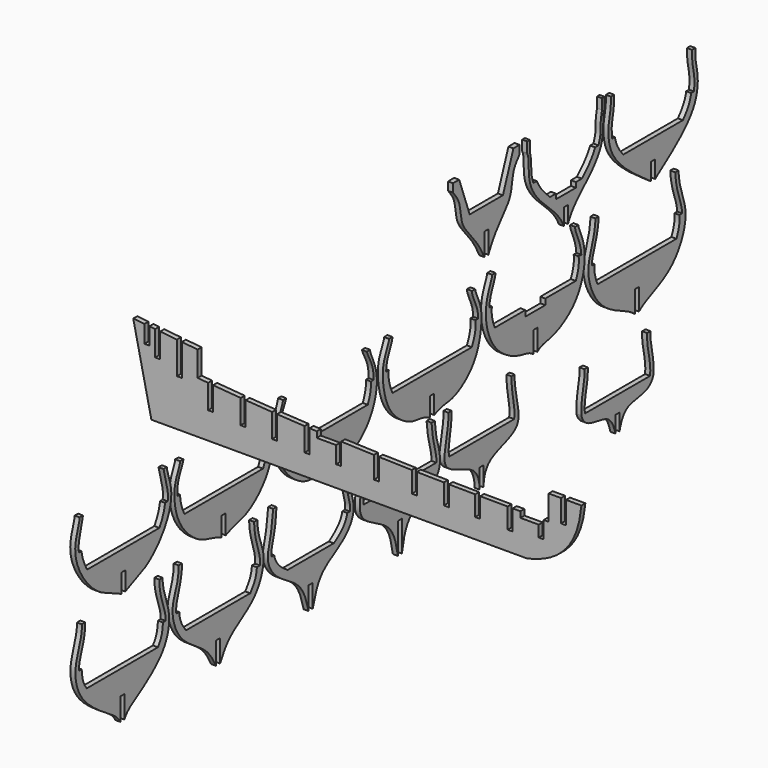
from build123d import *

# Parameters (mm, degrees)
F2_DEPTH = 6
F3_DEPTH = 6
F4_DEPTH = 6


# Not quite as in the source:
# - the dataset's text gives a spline's control points without its knots; the knots are read off the source's solid


with BuildPart() as f2:
    # F1 (on Front) → F2 (new body)
    with BuildSketch(Plane.XZ):
        with BuildLine():
            Line((-52.7647346169, 6.4092771036), (-52.7647346169, 27.4262808222))
            Line((-52.7647346169, 27.4262808222), (-66.1979233911, 28.7622259646))
            Line((-66.1979233911, 28.7622259646), (-44.4009490311, -71.2377740354))
            Line((-44.4009490311, -71.2377740354), (406.4361155033, -71.2503492832))
            add(Edge.make_bspline(
                [(472.4627340883, 6.0305400733), (469.2855259031, -29.0932188761), (455.8456540108, -61.0640123487), (406.4361155033, -71.2503492832)],
                knots=[0, 0, 0, 0, 101.6457093118, 101.6457093118, 101.6457093118, 101.6457093118], degree=3))
            Line((472.4627340883, 6.0305400733), (453.9572103575, 6.0305400733))
            Line((453.9572103575, 6.0305400733), (453.9572103575, -20.8669396024))
            Line((453.9572103575, -20.8669396024), (447.9572103575, -20.8669396024))
            Line((447.9572103575, -20.8669396024), (447.9572103575, 6.0305400733))
            Line((447.9572103575, 6.0305400733), (433.1729027743, 6.0305400733))
            Line((433.1729027743, 6.0305400733), (433.1729027743, -23.9694599267))
            Line((433.1729027743, -23.9694599267), (427.1729027743, -23.9694599267))
            Line((427.1729027743, -23.9694599267), (427.1729027743, -44.4963090949))
            Line((427.1729027743, -44.4963090949), (421.1729027743, -44.4963090949))
            Line((421.1729027743, -44.4963090949), (421.1729027743, -30.8844919416))
            Line((421.1729027743, -30.8844919416), (399.1729027743, -30.8844919416))
            Line((399.1729027743, -30.8844919416), (399.1729027743, -23.8844919416))
            add(Edge.make_bspline(
                [(389.837728412, -23.8556215321), (392.9609048209, -23.8660342773), (396.0726119054, -23.8755794708), (399.1729027743, -23.8844919416)],
                knots=[372.875417635, 372.875417635, 372.875417635, 372.875417635, 383.3713742335, 383.3713742335, 383.3713742335, 383.3713742335], degree=3))
            Line((389.837728412, -23.8556215321), (389.837728412, -48.3556215321))
            Line((389.837728412, -48.3556215321), (383.837728412, -48.3556215321))
            Line((383.837728412, -48.3556215321), (383.837728412, -23.8345407252))
            add(Edge.make_bspline(
                [(350.769388437, -23.667134025), (361.9320358553, -23.7417108378), (372.9540771428, -23.7942467699), (383.837728412, -23.8345407252)],
                knots=[329.7645780584, 329.7645780584, 329.7645780584, 329.7645780584, 366.1698310192, 366.1698310192, 366.1698310192, 366.1698310192], degree=3))
            Line((350.769388437, -23.667134025), (350.769388437, -47.6760274548))
            Line((350.769388437, -47.6760274548), (344.769388437, -47.6760274548))
            Line((344.769388437, -47.6760274548), (344.769388437, -23.6249695371))
            add(Edge.make_bspline(
                [(313.1183860302, -23.3244343777), (323.79185462, -23.4504439584), (334.3415946227, -23.5479952891), (344.769388437, -23.6249695371)],
                knots=[289.4005992863, 289.4005992863, 289.4005992863, 289.4005992863, 323.2565547842, 323.2565547842, 323.2565547842, 323.2565547842], degree=3))
            Line((313.1183860302, -23.3244343777), (313.1183860302, -47.6760274548))
            Line((313.1183860302, -47.6760274548), (307.1183860302, -47.6760274548))
            Line((307.1183860302, -47.6760274548), (307.1183860302, -23.2507163116))
            add(Edge.make_bspline(
                [(274.6596933386, -22.7436511652), (285.6039372317, -22.9476874536), (296.4229113646, -23.114099956), (307.1183860302, -23.2507163116)],
                knots=[249.2912534765, 249.2912534765, 249.2912534765, 249.2912534765, 283.0703857381, 283.0703857381, 283.0703857381, 283.0703857381], degree=3))
            Line((274.6596933386, -22.7436511652), (274.6596933386, -47.7436511652))
            Line((274.6596933386, -47.7436511652), (268.6600744313, -47.6760274548))
            Line((268.6600744313, -47.6760274548), (268.6600744313, -22.6282312507))
            add(Edge.make_bspline(
                [(229.0721806654, -21.6760274548), (242.4463483489, -22.0569030554), (255.6413320048, -22.3699669668), (268.6600744313, -22.6282312507)],
                knots=[203.116799722, 203.116799722, 203.116799722, 203.116799722, 243.1315638336, 243.1315638336, 243.1315638336, 243.1315638336], degree=3))
            Line((229.0721806654, -21.6760274548), (229.0721806654, -47.6760274548))
            Line((229.0721806654, -47.6760274548), (223.0721806654, -47.6760274548))
            Line((223.0721806654, -47.6760274548), (223.0721806654, -21.5009235146))
            add(Edge.make_bspline(
                [(183.718174545, -20.1332325707), (197.0050074387, -20.6617902502), (210.122129551, -21.1137964867), (223.0721806654, -21.5009235146)],
                knots=[158.5535490267, 158.5535490267, 158.5535490267, 158.5535490267, 197.1448620341, 197.1448620341, 197.1448620341, 197.1448620341], degree=3))
            Line((183.718174545, -20.1332325707), (183.718174545, -46.1332325707))
            Line((183.718174545, -46.1332325707), (177.718174545, -46.1332325707))
            Line((177.718174545, -46.1332325707), (177.718174545, -25.8504879718))
            Line((177.718174545, -25.8504879718), (154.3836850367, -25.8504879718))
            Line((154.3836850367, -25.8504879718), (154.3836850367, -18.8504879718))
            add(Edge.make_bspline(
                [(145.7038573316, -18.4253957008), (148.6049499698, -18.5710339991), (151.4982173473, -18.7126937317), (154.3836850367, -18.8504879718)],
                knots=[122.1894396031, 122.1894396031, 122.1894396031, 122.1894396031, 130.4161202076, 130.4161202076, 130.4161202076, 130.4161202076], degree=3))
            Line((145.7038573316, -18.4253957008), (145.7038573316, -46.1190585614))
            Line((145.7038573316, -46.1190585614), (139.7038573316, -46.1190585614))
            Line((139.7038573316, -46.1190585614), (139.7038573316, -18.1190585614))
            add(Edge.make_bspline(
                [(106.7340095181, -16.2487908881), (117.8343414661, -16.9327762992), (128.8238460829, -17.5542327451), (139.7038573316, -18.1190585614)],
                knots=[85.7901099469, 85.7901099469, 85.7901099469, 85.7901099469, 116.5285186795, 116.5285186795, 116.5285186795, 116.5285186795], degree=3))
            Line((106.7340095181, -16.2487908881), (106.7340095181, -44.4963090949))
            Line((106.7340095181, -44.4963090949), (100.7340095181, -44.4963090949))
            Line((100.7340095181, -44.4963090949), (100.7340095181, -15.8736411522))
            add(Edge.make_bspline(
                [(68.9865160879, -13.7047010206), (79.668117991, -14.4872744185), (90.2502452137, -15.2086158496), (100.7340095181, -15.8736411522)],
                knots=[51.3347121322, 51.3347121322, 51.3347121322, 51.3347121322, 80.2617577764, 80.2617577764, 80.2617577764, 80.2617577764], degree=3))
            Line((68.9865160879, -13.7047010206), (68.9865160879, -42.2594336062))
            Line((68.9865160879, -42.2594336062), (62.9865160879, -42.2594336062))
            Line((62.9865160879, -42.2594336062), (62.9865160879, -13.2594336062))
            add(Edge.make_bspline(
                [(29.770050062, -10.5860133059), (40.9473587591, -11.5457307631), (52.0191171292, -12.4351155869), (62.9865160879, -13.2594336062)],
                knots=[16.3300220537, 16.3300220537, 16.3300220537, 16.3300220537, 45.9278927601, 45.9278927601, 45.9278927601, 45.9278927601], degree=3))
            Line((29.770050062, -10.5860133059), (29.770050062, -39.0649404954))
            Line((29.770050062, -39.0649404954), (23.770050062, -39.0649404954))
            Line((23.770050062, -39.0649404954), (23.770050062, -10.0649404954))
            add(Edge.make_bspline(
                [(11.1729027743, -8.9323863213), (15.3867154839, -9.3200080517), (19.5857439628, -9.6974349483), (23.770050062, -10.0649404954)],
                knots=[0, 0, 0, 0, 11.0428828538, 11.0428828538, 11.0428828538, 11.0428828538], degree=3))
            Line((11.1729027743, -8.9323863213), (11.1729027743, 21.0676136787))
            Line((11.1729027743, 21.0676136787), (-7.7765522316, 22.95215746))
            Line((-7.7765522316, 22.95215746), (-7.7765522316, -15.2084504512))
            Line((-7.7765522316, -15.2084504512), (-13.7765522316, -15.2084504512))
            Line((-13.7765522316, -15.2084504512), (-13.7765522316, 23.5488639449))
            Line((-13.7765522316, 23.5488639449), (-33.8324046483, 25.5434401444))
            Line((-33.8324046483, 25.5434401444), (-33.8324046483, -3.8689912035))
            Line((-33.8324046483, -3.8689912035), (-39.8324046483, -3.8689912035))
            Line((-39.8324046483, -3.8689912035), (-39.8324046483, 26.1401466293))
            Line((-39.8324046483, 26.1401466293), (-46.7647346169, 26.8295743373))
            Line((-46.7647346169, 26.8295743373), (-46.7647346169, 6.4092771036))
            Line((-46.7647346169, 6.4092771036), (-52.7647346169, 6.4092771036))
        make_face()
    extrude(amount=F2_DEPTH)


with BuildPart() as f3:
    # F0 (on Right) → F3 (new body)
    with BuildSketch(Plane.YZ):
        with BuildLine():
            Line((484.2335848808, 26.7561373482), (484.2335848808, 36.7561373482))
            Line((484.2335848808, 36.7561373482), (474.9606251717, 36.7561373482))
            Line((474.9606251717, 36.7561373482), (459.2335848808, -6.4535507257))
            Line((459.2335848808, -6.4535507257), (434.2335848808, -6.4535507257))
            Line((434.2335848808, -6.4535507257), (409.2335848808, -6.4535507257))
            Line((409.2335848808, -6.4535507257), (393.50654459, 36.7561373482))
            Line((393.50654459, 36.7561373482), (384.2335848808, 36.7561373482))
            Line((384.2335848808, 36.7561373482), (384.2335848808, 26.7561373482))
            add(Edge.make_bspline(
                [(384.2335848808, 26.7561373482), (388.2177756268, 21.4898046256), (395.756738688, 13.2640159255), (394.9983547243, -19.9313208632), (418.2162308583, -32.7103473539), (431.2335848808, -60.5220484062)],
                knots=[0, 0, 0, 0, 0.2478083853, 0.549028575, 1, 1, 1, 1], degree=3))
            Line((431.2335848808, -60.5220484062), (431.2335848808, -33.4834151596))
            Line((431.2335848808, -33.4834151596), (437.2335848808, -33.4834151596))
            Line((437.2335848808, -33.4834151596), (437.2335848808, -60.5220484062))
            add(Edge.make_bspline(
                [(484.2335848808, 26.7561373482), (480.2493941349, 21.4898046256), (472.7104310736, 13.2640159255), (473.4688150374, -19.9313208632), (450.2509389033, -32.7103473539), (437.2335848808, -60.5220484062)],
                knots=[0, 0, 0, 0, 0.2478083853, 0.549028575, 1, 1, 1, 1], degree=3))
        make_face()
    extrude(amount=F3_DEPTH)

    # F0 (on Right) → F4 (join)
    with BuildSketch(Plane.YZ):
        with BuildLine():
            Line((484.2335848808, 26.7561373482), (484.2335848808, 36.7561373482))
            Line((484.2335848808, 36.7561373482), (474.9606251717, 36.7561373482))
            Line((474.9606251717, 36.7561373482), (459.2335848808, -6.4535507257))
            Line((459.2335848808, -6.4535507257), (434.2335848808, -6.4535507257))
            Line((434.2335848808, -6.4535507257), (409.2335848808, -6.4535507257))
            Line((409.2335848808, -6.4535507257), (393.50654459, 36.7561373482))
            Line((393.50654459, 36.7561373482), (384.2335848808, 36.7561373482))
            Line((384.2335848808, 36.7561373482), (384.2335848808, 26.7561373482))
            add(Edge.make_bspline(
                [(384.2335848808, 26.7561373482), (388.2177756268, 21.4898046256), (395.756738688, 13.2640159255), (394.9983547243, -19.9313208632), (418.2162308583, -32.7103473539), (431.2335848808, -60.5220484062)],
                knots=[0, 0, 0, 0, 0.2478083853, 0.549028575, 1, 1, 1, 1], degree=3))
            Line((431.2335848808, -60.5220484062), (431.2335848808, -33.4834151596))
            Line((431.2335848808, -33.4834151596), (437.2335848808, -33.4834151596))
            Line((437.2335848808, -33.4834151596), (437.2335848808, -60.5220484062))
            add(Edge.make_bspline(
                [(484.2335848808, 26.7561373482), (480.2493941349, 21.4898046256), (472.7104310736, 13.2640159255), (473.4688150374, -19.9313208632), (450.2509389033, -32.7103473539), (437.2335848808, -60.5220484062)],
                knots=[0, 0, 0, 0, 0.2478083853, 0.549028575, 1, 1, 1, 1], degree=3))
        make_face()
    extrude(amount=F4_DEPTH)


with BuildPart() as f4:
    # F0 (on Right) → F4, piece 2 (new body)
    with BuildSketch(Plane.YZ):
        with BuildLine():
            Line((550.8763999939, -56.434545666), (553.8763999939, -56.434545666))
            Line((553.8763999939, -56.434545666), (556.8763999939, -56.434545666))
            Line((556.8763999939, -56.434545666), (556.8763999939, -76.434545666))
            add(Edge.make_bspline(
                [(612.0403327942, 23.1877360493), (610.674738884, 20.2818345279), (609.5481146502, 12.5812319025), (610.7848200662, -16.7130586961), (581.0642364303, -47.7261486798), (563.6113171122, -61.7929375305), (556.8763999939, -76.434545666)],
                knots=[0, 0, 0, 0, 0.152021729, 0.3997620662, 0.7016972465, 1, 1, 1, 1], degree=3))
            Line((612.0403327942, 23.1877360493), (612.0403327942, 35.6877360493))
            Line((612.0403327942, 35.6877360493), (608.0403327942, 35.6877360493))
            Line((608.0403327942, 35.6877360493), (608.0403327942, 23.1877360493))
            add(Edge.make_bspline(
                [(602.7448821068, -12.0413303375), (603.750125951, -8.9215364764), (606.3474615411, -2.2715853679), (605.6387899895, 10.3550530673), (606.7486405373, 17.3133779317), (608.0403327942, 23.1877360493)],
                knots=[0, 0, 0, 0, 0.3098493609, 0.6418818036, 1, 1, 1, 1], degree=3))
            Line((602.7448821068, -12.0413303375), (597.7448821068, -12.0413303375))
            add(Edge.make_bspline(
                [(577.8763999939, -37.0800281465), (586.0707759857, -29.3217152357), (592.6425457001, -22.6697772741), (597.7448821068, -12.0413303375)],
                knots=[0, 0, 0, 0, 31.9639323213, 31.9639323213, 31.9639323213, 31.9639323213], degree=3))
            Line((577.8763999939, -37.0800281465), (568.8763999939, -37.0800281465))
            Line((568.8763999939, -37.0800281465), (568.8763999939, -43.0800281465))
            Line((568.8763999939, -43.0800281465), (553.8763999939, -43.0800281465))
            Line((553.8763999939, -43.0800281465), (538.8763999939, -43.0800281465))
            Line((538.8763999939, -43.0800281465), (538.8763999939, -37.0800281465))
            Line((538.8763999939, -37.0800281465), (529.8763999939, -37.0800281465))
            add(Edge.make_bspline(
                [(529.8763999939, -37.0800281465), (521.6820240021, -29.3217152357), (515.1102542877, -22.6697772741), (510.007917881, -12.0413303375)],
                knots=[0, 0, 0, 0, 31.9639323213, 31.9639323213, 31.9639323213, 31.9639323213], degree=3))
            Line((510.007917881, -12.0413303375), (505.007917881, -12.0413303375))
            add(Edge.make_bspline(
                [(505.007917881, -12.0413303375), (504.0026740368, -8.9215364764), (501.4053384467, -2.2715853679), (502.1140099983, 10.3550530673), (501.0041594505, 17.3133779317), (499.7124671936, 23.1877360493)],
                knots=[0, 0, 0, 0, 0.3098493609, 0.6418818036, 1, 1, 1, 1], degree=3))
            Line((499.7124671936, 23.1877360493), (499.7124671936, 35.6877360493))
            Line((499.7124671936, 35.6877360493), (495.7124671936, 35.6877360493))
            Line((495.7124671936, 35.6877360493), (495.7124671936, 23.1877360493))
            add(Edge.make_bspline(
                [(495.7124671936, 23.1877360493), (497.0780611038, 20.2818345279), (498.2046853376, 12.5812319025), (496.9679799216, -16.7130586961), (526.6885635575, -47.7261486798), (544.1414828756, -61.7929375305), (550.8763999939, -76.434545666)],
                knots=[0, 0, 0, 0, 0.152021729, 0.3997620662, 0.7016972465, 1, 1, 1, 1], degree=3))
            Line((550.8763999939, -76.434545666), (550.8763999939, -56.434545666))
        make_face()
    extrude(amount=F4_DEPTH)


with BuildPart() as f4b:
    # F0 (on Right) → F4, piece 3 (new body)
    with BuildSketch(Plane.YZ):
        with BuildLine():
            Line((628.2879323959, -307.473314481), (631.2879323959, -307.473314481))
            Line((631.2879323959, -307.473314481), (634.2879323959, -307.473314481))
            Line((634.2879323959, -307.473314481), (634.2879323959, -327.473314481))
            add(Edge.make_bspline(
                [(685.2788976234, -287.6933656511), (685.1189731977, -290.2255342926), (678.5230453699, -304.1369421605), (642.1088001808, -301.8919192623), (636.5011588194, -319.6582646749), (634.2879323959, -327.473314481)],
                knots=[0, 0, 0, 0, 0.26107974, 0.6603595506, 1, 1, 1, 1], degree=3))
            add(Edge.make_bspline(
                [(685.2788976234, -287.6933656511), (685.5841961705, -285.0556549193), (685.7341073494, -279.7660437072), (685.1329208416, -273.4266273945), (684.3904637761, -268.5638979594), (683.758391527, -265.0694275356), (683.10342587, -261.7522406842), (682.4767926926, -258.6421978218), (682.0192982988, -256.2487303118), (681.7169724365, -254.4812661897), (681.4602613553, -252.7979998546), (681.213445371, -250.8086895139), (681.0190368897, -248.574522162), (680.9085692934, -246.4483229789), (680.8520494131, -243.7120175126), (680.8881439051, -241.6960916439), (680.927080808, -240.3208393524)],
                knots=[0.0030955746, 0.0030955746, 0.0030955746, 0.0030955746, 0.125, 0.25, 0.3125, 0.375, 0.4375, 0.5, 0.5625, 0.59375, 0.625, 0.6875, 0.75, 0.8125, 0.875, 0.9990042973, 0.9990042973, 0.9990042973, 0.9990042973], degree=3))
            Line((680.927080808, -240.3208393524), (675.927080808, -240.3208393524))
            add(Edge.make_bspline(
                [(680.2879323959, -287.473314481), (681.6616019621, -276.0409791318), (675.846007472, -256.1593083122), (675.7951415299, -244.9544503514), (675.927080808, -240.3208393524)],
                knots=[0, 0, 0, 0, 0.5921365734, 1, 1, 1, 1], degree=3))
            Line((680.2879323959, -287.473314481), (631.2879323959, -287.473314481))
            Line((631.2879323959, -287.473314481), (582.2879323959, -287.473314481))
            add(Edge.make_bspline(
                [(582.2879323959, -287.473314481), (580.9142628298, -276.0409791318), (586.7298573198, -256.1593083122), (586.780723262, -244.9544503514), (586.6487839839, -240.3208393524)],
                knots=[0, 0, 0, 0, 0.5921365734, 1, 1, 1, 1], degree=3))
            Line((586.6487839839, -240.3208393524), (581.6487839839, -240.3208393524))
            add(Edge.make_bspline(
                [(577.2969671685, -287.6933656511), (576.9916686214, -285.0556549193), (576.8417574425, -279.7660437072), (577.4429439503, -273.4266273945), (578.1854010158, -268.5638979594), (578.8174732648, -265.0694275356), (579.4724389219, -261.7522406842), (580.0990720993, -258.6421978218), (580.556566493, -256.2487303118), (580.8588923554, -254.4812661897), (581.1156034366, -252.7979998546), (581.3624194209, -250.8086895139), (581.5568279022, -248.574522162), (581.6672954985, -246.4483229789), (581.7238153788, -243.7120175126), (581.6877208868, -241.6960916439), (581.6487839839, -240.3208393524)],
                knots=[0.0030955746, 0.0030955746, 0.0030955746, 0.0030955746, 0.125, 0.25, 0.3125, 0.375, 0.4375, 0.5, 0.5625, 0.59375, 0.625, 0.6875, 0.75, 0.8125, 0.875, 0.9990042973, 0.9990042973, 0.9990042973, 0.9990042973], degree=3))
            add(Edge.make_bspline(
                [(577.2969671685, -287.6933656511), (577.4568915941, -290.2255342926), (584.0528194219, -304.1369421605), (620.4670646111, -301.8919192623), (626.0747059724, -319.6582646749), (628.2879323959, -327.473314481)],
                knots=[0, 0, 0, 0, 0.26107974, 0.6603595506, 1, 1, 1, 1], degree=3))
            Line((628.2879323959, -327.473314481), (628.2879323959, -307.473314481))
        make_face()
    extrude(amount=F4_DEPTH)


with BuildPart() as f4c:
    # F0 (on Right) → F4, piece 4 (new body)
    with BuildSketch(Plane.YZ):
        with BuildLine():
            Line((424.0916283131, -280.193121695), (427.0916283131, -280.193121695))
            Line((427.0916283131, -280.193121695), (430.0916283131, -280.193121695))
            Line((430.0916283131, -280.193121695), (430.0916283131, -303.6715098868))
            add(Edge.make_bspline(
                [(476.915219004, -203.2369971275), (475.5835916351, -224.0514308214), (499.1814730372, -266.8526601855), (432.7437947726, -272.5029182243), (430.0916283131, -297.2647651872), (430.0916283131, -303.6715098868)],
                knots=[0, 0, 0, 0, 0.3847055744, 0.7392693423, 1, 1, 1, 1], degree=3))
            Line((476.915219004, -203.2369971275), (471.915219004, -203.2369971275))
            add(Edge.make_bspline(
                [(476.0916283131, -250.193121695), (477.1469744668, -241.4100260832), (474.8519464487, -233.504609702), (471.7388915262, -209.4294892532), (471.915219004, -203.2369971275)],
                knots=[0, 0, 0, 0, 0.4549194876, 1, 1, 1, 1], degree=3))
            Line((476.0916283131, -250.193121695), (427.0916283131, -250.193121695))
            Line((427.0916283131, -250.193121695), (378.0916283131, -250.193121695))
            add(Edge.make_bspline(
                [(378.0916283131, -250.193121695), (377.0362821593, -241.4100260832), (379.3313101774, -233.504609702), (382.4443650999, -209.4294892532), (382.2680376221, -203.2369971275)],
                knots=[0, 0, 0, 0, 0.4549194876, 1, 1, 1, 1], degree=3))
            Line((382.2680376221, -203.2369971275), (377.2680376221, -203.2369971275))
            add(Edge.make_bspline(
                [(377.2680376221, -203.2369971275), (378.5996649911, -224.0514308214), (355.0017835889, -266.8526601855), (421.4394618535, -272.5029182243), (424.0916283131, -297.2647651872), (424.0916283131, -303.6715098868)],
                knots=[0, 0, 0, 0, 0.3847055744, 0.7392693423, 1, 1, 1, 1], degree=3))
            Line((424.0916283131, -303.6715098868), (424.0916283131, -280.193121695))
        make_face()
    extrude(amount=F4_DEPTH)


with BuildPart() as f4d:
    # F0 (on Right) → F4, piece 5 (new body)
    with BuildSketch(Plane.YZ):
        with BuildLine():
            Line((301.3534755707, -286.9323194027), (304.3534755707, -286.9323194027))
            Line((304.3534755707, -286.9323194027), (307.3534755707, -286.9323194027))
            Line((307.3534755707, -286.9323194027), (307.3534755707, -323.9323194027))
            add(Edge.make_bspline(
                [(307.3534755707, -323.9323194027), (309.7463144575, -310.4888525345), (315.1184452247, -281.9415644206), (371.7815140601, -267.3580642044), (363.8714849949, -237.3508810997), (359.8218560219, -224.1371721029)],
                knots=[0, 0, 0, 0, 0.3276113271, 0.6831504771, 1, 1, 1, 1], degree=3))
            add(Edge.make_bspline(
                [(359.8218560219, -224.1371721029), (358.1883907318, -217.5396382809), (357.8812479973, -210.4500979185), (356.9385707378, -203.5875618458)],
                knots=[0, 0, 0, 0, 20.7508991552, 20.7508991552, 20.7508991552, 20.7508991552], degree=3))
            Line((356.9385707378, -203.5875618458), (351.9385707378, -203.5875618458))
            add(Edge.make_bspline(
                [(351.9385707378, -203.5875618458), (353.2665371895, -216.3607180119), (354.040820554, -222.3392811996), (359.9659204483, -243.4709519148), (359.1620028019, -248.7411499023)],
                knots=[0, 0, 0, 0, 0.4988788112, 1, 1, 1, 1], degree=3))
            Line((359.1620028019, -248.7411499023), (304.3534755707, -248.7411499023))
            Line((304.3534755707, -248.7411499023), (249.5449483395, -248.7411499023))
            add(Edge.make_bspline(
                [(256.7683804035, -203.5875618458), (255.4404139519, -216.3607180119), (254.6661305873, -222.3392811996), (248.7410306931, -243.4709519148), (249.5449483395, -248.7411499023)],
                knots=[0, 0, 0, 0, 0.4988788112, 1, 1, 1, 1], degree=3))
            Line((256.7683804035, -203.5875618458), (251.7683804035, -203.5875618458))
            add(Edge.make_bspline(
                [(248.8850951195, -224.1371721029), (250.5185604095, -217.5396382809), (250.8257031441, -210.4500979185), (251.7683804035, -203.5875618458)],
                knots=[0, 0, 0, 0, 20.7508991552, 20.7508991552, 20.7508991552, 20.7508991552], degree=3))
            add(Edge.make_bspline(
                [(301.3534755707, -323.9323194027), (298.9606366838, -310.4888525345), (293.5885059166, -281.9415644206), (236.9254370813, -267.3580642044), (244.8354661465, -237.3508810997), (248.8850951195, -224.1371721029)],
                knots=[0, 0, 0, 0, 0.3276113271, 0.6831504771, 1, 1, 1, 1], degree=3))
            Line((301.3534755707, -323.9323194027), (301.3534755707, -286.9323194027))
        make_face()
    extrude(amount=F4_DEPTH)


with BuildPart() as f4e:
    # F0 (on Right) → F4, piece 6 (new body)
    with BuildSketch(Plane.YZ):
        with BuildLine():
            Line((167.4125851393, -300.40538311), (170.4125851393, -300.40538311))
            Line((170.4125851393, -300.40538311), (173.4125851393, -300.40538311))
            Line((173.4125851393, -300.40538311), (173.4125851393, -327.90538311))
            add(Edge.make_bspline(
                [(173.4125851393, -327.90538311), (176.6649784086, -316.0511091836), (183.3397189291, -291.7852840199), (223.3479008677, -275.2949217188), (238.2419790008, -248.8329841394), (230.1760505039, -227.1787029617), (228.0389055604, -208.7248289279), (226.8404662609, -197.9364901781)],
                knots=[0, 0, 0, 0, 0.2157693607, 0.447354947, 0.6349702267, 0.8018901494, 1, 1, 1, 1], degree=3))
            Line((226.8404662609, -197.9364901781), (221.8404662609, -197.9364901781))
            add(Edge.make_bspline(
                [(221.8404662609, -197.9364901781), (222.4405672875, -206.113414408), (223.5184825579, -222.3151099473), (230.3157597537, -239.526123779), (229.4610350683, -247.0080951132), (229.3689863855, -247.5943883923)],
                knots=[0, 0, 0, 0, 0.3552465033, 0.70211507, 0.7320300869, 0.7320300869, 0.7320300869, 0.7320300869], degree=3))
            Line((229.3689863855, -247.5943883923), (225.3689863855, -247.5943883923))
            add(Edge.make_bspline(
                [(225.3689863855, -247.5943883923), (223.0493873358, -258.7058246136), (214.3388241529, -265.6163117886), (205.0644784033, -271.40538311)],
                knots=[0, 0, 0, 0, 31.2927549737, 31.2927549737, 31.2927549737, 31.2927549737], degree=3))
            Line((205.0644784033, -271.40538311), (170.4125851393, -271.40538311))
            Line((170.4125851393, -271.40538311), (135.7606918752, -271.40538311))
            add(Edge.make_bspline(
                [(115.4561838931, -247.5943883923), (117.7757829428, -258.7058246136), (126.4863461256, -265.6163117886), (135.7606918752, -271.40538311)],
                knots=[0, 0, 0, 0, 31.2927549737, 31.2927549737, 31.2927549737, 31.2927549737], degree=3))
            Line((115.4561838931, -247.5943883923), (111.4561838931, -247.5943883923))
            add(Edge.make_bspline(
                [(118.9847040176, -197.9364901781), (118.3846029911, -206.113414408), (117.3066877207, -222.3151099473), (110.5094105249, -239.526123779), (111.3641352103, -247.0080951132), (111.4561838931, -247.5943883923)],
                knots=[0, 0, 0, 0, 0.3552465033, 0.70211507, 0.7320300869, 0.7320300869, 0.7320300869, 0.7320300869], degree=3))
            Line((118.9847040176, -197.9364901781), (113.9847040176, -197.9364901781))
            add(Edge.make_bspline(
                [(167.4125851393, -327.90538311), (164.1601918699, -316.0511091836), (157.4854513495, -291.7852840199), (117.4772694109, -275.2949217188), (102.5831912778, -248.8329841394), (110.6491197747, -227.1787029617), (112.7862647181, -208.7248289279), (113.9847040176, -197.9364901781)],
                knots=[0, 0, 0, 0, 0.2157693607, 0.447354947, 0.6349702267, 0.8018901494, 1, 1, 1, 1], degree=3))
            Line((167.4125851393, -327.90538311), (167.4125851393, -300.40538311))
        make_face()
    extrude(amount=F4_DEPTH)


with BuildPart() as f4f:
    # F0 (on Right) → F4, piece 7 (new body)
    with BuildSketch(Plane.YZ):
        with BuildLine():
            Line((28.2110185623, -302.2633194923), (31.2110185623, -302.2633194923))
            Line((31.2110185623, -302.2633194923), (34.2110185623, -302.2633194923))
            Line((34.2110185623, -302.2633194923), (34.2110185623, -329.2633194923))
            add(Edge.make_bspline(
                [(34.2110185623, -329.2633194923), (38.4308069632, -321.3498655437), (47.9631956452, -303.2676923795), (90.8464226956, -283.7047870015), (103.2311789873, -243.0394325924), (93.3035786994, -223.3674999276), (90.1412684486, -206.9374462595), (90.3983238339, -200.0559866428)],
                knots=[0, 0, 0, 0, 0.191927042, 0.4362269972, 0.6591727134, 0.8274439614, 1, 1, 1, 1], degree=3))
            Line((90.3983238339, -200.0559866428), (85.3983238339, -200.0559866428))
            add(Edge.make_bspline(
                [(85.3983238339, -200.0559866428), (85.3551956512, -208.1565379637), (88.6282257993, -224.7674824207), (94.9553428478, -239.7215619517), (94.0034165978, -249.7978359461)],
                knots=[0, 0, 0, 0, 0.4909376569, 1, 1, 1, 1], degree=3))
            Line((94.0034165978, -249.7978359461), (89.5419120789, -249.7978359461))
            add(Edge.make_bspline(
                [(79.5613378286, -273.2633194923), (84.3899324536, -266.581594944), (88.692098856, -261.3765001297), (89.5419120789, -249.7978359461)],
                knots=[0, 0, 0, 0, 25.4998192234, 25.4998192234, 25.4998192234, 25.4998192234], degree=3))
            Line((79.5613378286, -273.2633194923), (31.2110185623, -273.2633194923))
            Line((31.2110185623, -273.2633194923), (-17.139300704, -273.2633194923))
            add(Edge.make_bspline(
                [(-17.139300704, -273.2633194923), (-21.967895329, -266.581594944), (-26.2700617313, -261.3765001297), (-27.1198749542, -249.7978359461)],
                knots=[0, 0, 0, 0, 25.4998192234, 25.4998192234, 25.4998192234, 25.4998192234], degree=3))
            Line((-27.1198749542, -249.7978359461), (-31.5813794732, -249.7978359461))
            add(Edge.make_bspline(
                [(-22.9762867093, -200.0559866428), (-22.9331585266, -208.1565379637), (-26.2061886747, -224.7674824207), (-32.5333057232, -239.7215619517), (-31.5813794732, -249.7978359461)],
                knots=[0, 0, 0, 0, 0.4909376569, 1, 1, 1, 1], degree=3))
            Line((-22.9762867093, -200.0559866428), (-27.9762867093, -200.0559866428))
            add(Edge.make_bspline(
                [(28.2110185623, -329.2633194923), (23.9912301614, -321.3498655437), (14.4588414794, -303.2676923795), (-28.4243855709, -283.7047870015), (-40.8091418626, -243.0394325924), (-30.8815415748, -223.3674999276), (-27.719231324, -206.9374462595), (-27.9762867093, -200.0559866428)],
                knots=[0, 0, 0, 0, 0.191927042, 0.4362269972, 0.6591727134, 0.8274439614, 1, 1, 1, 1], degree=3))
            Line((28.2110185623, -329.2633194923), (28.2110185623, -302.2633194923))
        make_face()
    extrude(amount=F4_DEPTH)


with BuildPart() as f4g:
    # F0 (on Right) → F4, piece 8 (new body)
    with BuildSketch(Plane.YZ):
        with BuildLine():
            Line((-115.6893894076, -303.0414440632), (-112.6893894076, -303.0414440632))
            Line((-112.6893894076, -303.0414440632), (-109.6893894076, -303.0414440632))
            Line((-109.6893894076, -303.0414440632), (-109.6893894076, -330.0414440632))
            add(Edge.make_bspline(
                [(-109.6893894076, -330.0414440632), (-105.4760691243, -322.1401199054), (-87.8114329254, -312.1269073727), (-47.901149894, -284.560894306), (-39.1369988781, -248.3245994379), (-49.1970523964, -224.1850619521), (-52.2715479042, -209.8299341498), (-52.0269796252, -203.2827585936)],
                knots=[0, 0, 0, 0, 0.1916328551, 0.4414824997, 0.653540961, 0.8358263012, 1, 1, 1, 1], degree=3))
            Line((-52.0269796252, -203.2827585936), (-57.0269796252, -203.2827585936))
            add(Edge.make_bspline(
                [(-57.0269796252, -203.2827585936), (-57.0701741706, -211.395774471), (-54.1319871103, -227.0575896721), (-47.4235753985, -241.0529633111), (-47.6227968037, -250.7734596729)],
                knots=[0, 0, 0, 0, 0.4916930771, 1, 1, 1, 1], degree=3))
            Line((-47.6227968037, -250.7734596729), (-51.6227968037, -250.7734596729))
            add(Edge.make_bspline(
                [(-59.1654218733, -274.0414440632), (-54.3368272483, -267.3597195148), (-52.4726100266, -262.3521238565), (-51.6227968037, -250.7734596729)],
                knots=[0, 0, 0, 0, 24.4599732323, 24.4599732323, 24.4599732323, 24.4599732323], degree=3))
            Line((-59.1654218733, -274.0414440632), (-112.6893894076, -274.0414440632))
            Line((-112.6893894076, -274.0414440632), (-166.2133569419, -274.0414440632))
            add(Edge.make_bspline(
                [(-166.2133569419, -274.0414440632), (-171.0419515669, -267.3597195148), (-172.9061687887, -262.3521238565), (-173.7559820116, -250.7734596729)],
                knots=[0, 0, 0, 0, 24.4599732323, 24.4599732323, 24.4599732323, 24.4599732323], degree=3))
            Line((-173.7559820116, -250.7734596729), (-177.7559820116, -250.7734596729))
            add(Edge.make_bspline(
                [(-168.35179919, -203.2827585936), (-168.3086046447, -211.395774471), (-171.246791705, -227.0575896721), (-177.9552034168, -241.0529633111), (-177.7559820116, -250.7734596729)],
                knots=[0, 0, 0, 0, 0.4916930771, 1, 1, 1, 1], degree=3))
            Line((-168.35179919, -203.2827585936), (-173.35179919, -203.2827585936))
            add(Edge.make_bspline(
                [(-115.6893894076, -330.0414440632), (-119.9027096909, -322.1401199054), (-137.5673458899, -312.1269073727), (-177.4776289213, -284.560894306), (-186.2417799371, -248.3245994379), (-176.1817264189, -224.1850619521), (-173.107230911, -209.8299341498), (-173.35179919, -203.2827585936)],
                knots=[0, 0, 0, 0, 0.1916328551, 0.4414824997, 0.653540961, 0.8358263012, 1, 1, 1, 1], degree=3))
            Line((-115.6893894076, -330.0414440632), (-115.6893894076, -303.0414440632))
        make_face()
    extrude(amount=F4_DEPTH)


with BuildPart() as f4h:
    # F0 (on Right) → F4, piece 9 (new body)
    with BuildSketch(Plane.YZ):
        with BuildLine():
            Line((657.6085300446, -186.4504111489), (660.6085300446, -186.4504111489))
            Line((660.6085300446, -186.4504111489), (663.6085300446, -186.4504111489))
            Line((663.6085300446, -186.4504111489), (663.6085300446, -212.6357257366))
            add(Edge.make_bspline(
                [(663.6085300446, -212.6357257366), (669.6908238858, -207.5922178562), (684.2574754697, -201.0889348861), (719.2787469814, -185.1408431756), (739.8064731312, -139.1409414867), (724.8986617241, -109.5291145707), (723.0969071594, -91.1269778126), (723.0969071594, -87.439360776)],
                knots=[0, 0, 0, 0, 0.1730259257, 0.3920092663, 0.6340960494, 0.8403459133, 1, 1, 1, 1], degree=3))
            Line((723.0969071594, -87.439360776), (718.0969071594, -87.439360776))
            add(Edge.make_bspline(
                [(728.5162643173, -135.1442276227), (728.4923331209, -134.7184067348), (728.4044417091, -133.5201280334), (728.1711653307, -131.567451637), (727.6437144958, -128.5229403361), (726.7173045751, -124.7315522578), (725.2998869861, -120.138049263), (723.9795053556, -116.2265633883), (722.917791077, -113.0179292084), (722.140236172, -110.5633140581), (721.4030388116, -108.054895656), (720.7315875724, -105.4763310451), (720.1524274056, -102.9117412059), (719.4876011525, -99.536180919), (718.8467831983, -95.4663755084), (718.3437852247, -91.0549790606), (718.1578162508, -88.5486569837), (718.0969071594, -87.439360776)],
                knots=[0.6476893065, 0.6476893065, 0.6476893065, 0.6476893065, 0.65625, 0.671875, 0.6875, 0.71875, 0.75, 0.78125, 0.796875, 0.8125, 0.828125, 0.84375, 0.859375, 0.875, 0.90625, 0.9375, 0.9681616833, 0.9681616833, 0.9681616833, 0.9681616833], degree=3))
            Line((728.5162643173, -135.1442276227), (724.5162643173, -135.1442276227))
            add(Edge.make_bspline(
                [(719.8877004438, -158.4504111489), (720.5174738825, -157.0634784211), (721.7831312494, -153.9867078113), (723.2937275194, -149.2398480195), (724.1597302529, -145.1857670033), (724.5595228465, -142.100176332), (724.7125658913, -139.8883329803), (724.7198716493, -137.7928708303), (724.6237068736, -136.2158315304), (724.5365023999, -135.3337134374), (724.5162643173, -135.1442276227)],
                knots=[0.5051635569, 0.5051635569, 0.5051635569, 0.5051635569, 0.53125, 0.5625, 0.59375, 0.609375, 0.625, 0.640625, 0.65625, 0.6605245417, 0.6605245417, 0.6605245417, 0.6605245417], degree=3))
            Line((719.8877004438, -158.4504111489), (660.6085300446, -158.4504111489))
            Line((660.6085300446, -158.4504111489), (601.3293596453, -158.4504111489))
            add(Edge.make_bspline(
                [(601.3293596453, -158.4504111489), (600.6995862066, -157.0634784211), (599.4339288397, -153.9867078113), (597.9233325697, -149.2398480195), (597.0573298362, -145.1857670033), (596.6575372426, -142.100176332), (596.5044941978, -139.8883329803), (596.4971884398, -137.7928708303), (596.5933532155, -136.2158315304), (596.6805576892, -135.3337134374), (596.7007957718, -135.1442276227)],
                knots=[0.5051635569, 0.5051635569, 0.5051635569, 0.5051635569, 0.53125, 0.5625, 0.59375, 0.609375, 0.625, 0.640625, 0.65625, 0.6605245417, 0.6605245417, 0.6605245417, 0.6605245417], degree=3))
            Line((596.7007957718, -135.1442276227), (592.7007957718, -135.1442276227))
            add(Edge.make_bspline(
                [(592.7007957718, -135.1442276227), (592.7247269682, -134.7184067348), (592.81261838, -133.5201280334), (593.0458947584, -131.567451637), (593.5733455933, -128.5229403361), (594.499755514, -124.7315522578), (595.917173103, -120.138049263), (597.2375547336, -116.2265633883), (598.2992690121, -113.0179292084), (599.0768239171, -110.5633140582), (599.8140212775, -108.054895656), (600.4854725167, -105.4763310451), (601.0646326835, -102.9117412059), (601.7294589366, -99.5361809191), (602.3702768908, -95.4663755084), (602.8732748645, -91.0549790607), (603.0592438383, -88.5486569837), (603.1201529298, -87.439360776)],
                knots=[0.6476893065, 0.6476893065, 0.6476893065, 0.6476893065, 0.65625, 0.671875, 0.6875, 0.71875, 0.75, 0.78125, 0.796875, 0.8125, 0.828125, 0.84375, 0.859375, 0.875, 0.90625, 0.9375, 0.9681616833, 0.9681616833, 0.9681616833, 0.9681616833], degree=3))
            Line((603.1201529298, -87.439360776), (598.1201529298, -87.439360776))
            add(Edge.make_bspline(
                [(657.6085300446, -212.6357257366), (651.5262362034, -207.5922178562), (636.9595846194, -201.0889348861), (601.9383131077, -185.1408431756), (581.4105869579, -139.1409414867), (596.318398365, -109.5291145707), (598.1201529298, -91.1269778126), (598.1201529298, -87.439360776)],
                knots=[0, 0, 0, 0, 0.1730259257, 0.3920092663, 0.6340960494, 0.8403459133, 1, 1, 1, 1], degree=3))
            Line((657.6085300446, -212.6357257366), (657.6085300446, -186.4504111489))
        make_face()
    extrude(amount=F4_DEPTH)


with BuildPart() as f4i:
    # F0 (on Right) → F4, piece 10 (new body)
    with BuildSketch(Plane.YZ):
        with BuildLine():
            Line((504.8143687248, -167.5871324778), (507.8143687248, -167.5871324778))
            Line((507.8143687248, -167.5871324778), (510.8143687248, -167.5871324778))
            Line((510.8143687248, -167.5871324778), (510.8143687248, -193.1871324778))
            add(Edge.make_bspline(
                [(510.8143687248, -193.1871324778), (517.1117106988, -187.9653042168), (533.7992577613, -188.2154526704), (568.6612634985, -169.0143192502), (584.1136824409, -132.6547521793), (581.1204733465, -102.7194419017), (572.6380934566, -87.6802871123), (572.6380934566, -83.9864537864)],
                knots=[0, 0, 0, 0, 0.1791435029, 0.4065737207, 0.6352421206, 0.8400767813, 1, 1, 1, 1], degree=3))
            Line((572.6380934566, -83.9864537864), (567.6380934566, -83.9864537864))
            add(Edge.make_bspline(
                [(576.9884732479, -117.2925392224), (576.9269777761, -116.4915439883), (576.7081038409, -114.2700442071), (576.2501354965, -111.3822123744), (575.6575319077, -108.6307765289), (575.1416600615, -106.5961888273), (574.6543934758, -104.9271867011), (574.2314301384, -103.6089022635), (573.7869026819, -102.3034124691), (573.1848456362, -100.6684754723), (572.1575482864, -98.0711616981), (570.8147746676, -94.890094865), (569.5593026181, -91.8564883225), (568.7049540542, -89.5025937701), (568.1660843781, -87.7479841778), (567.7660623849, -85.9552945442), (567.6380934566, -84.6715799484), (567.6380934566, -83.9864537864)],
                knots=[0.7325128492, 0.7325128492, 0.7325128492, 0.7325128492, 0.75, 0.78125, 0.796875, 0.8125, 0.828125, 0.8359375, 0.84375, 0.859375, 0.875, 0.90625, 0.9375, 0.953125, 0.96875, 0.984375, 1, 1, 1, 1], degree=3))
            Line((576.9884732479, -117.2925392224), (572.9884732479, -117.2925392224))
            add(Edge.make_bspline(
                [(568.6603665013, -141.5871324778), (569.2361027896, -140.3011589832), (570.4497671347, -137.3281467772), (571.9274375745, -132.6847522875), (572.793440308, -128.6306712713), (573.1932329016, -125.5450805999), (573.3462759464, -123.3332372483), (573.3535817045, -121.2377750982), (573.2310394031, -119.2281616652), (573.0768163224, -117.9150315182), (572.9884732479, -117.2925392224)],
                knots=[0.5070944382, 0.5070944382, 0.5070944382, 0.5070944382, 0.53125, 0.5625, 0.59375, 0.609375, 0.625, 0.640625, 0.65625, 0.670268749, 0.670268749, 0.670268749, 0.670268749], degree=3))
            Line((568.6603665012, -141.5871324778), (522.8143687248, -141.5871324778))
            Line((522.8143687248, -141.5871324778), (522.8143687248, -148.5871324778))
            Line((522.8143687248, -148.5871324778), (507.8143687248, -148.5871324778))
            Line((507.8143687248, -148.5871324778), (492.8143687248, -148.5871324778))
            Line((492.8143687248, -148.5871324778), (492.8143687248, -141.5871324778))
            Line((492.8143687248, -141.5871324778), (446.9683709484, -141.5871324778))
            add(Edge.make_bspline(
                [(446.9683709484, -141.5871324778), (446.3926346601, -140.3011589832), (445.178970315, -137.3281467772), (443.7012998751, -132.6847522875), (442.8352971416, -128.6306712713), (442.435504548, -125.5450805999), (442.2824615033, -123.3332372483), (442.2751557452, -121.2377750982), (442.3976980465, -119.2281616652), (442.5519211273, -117.9150315182), (442.6402642018, -117.2925392225)],
                knots=[0.5070944382, 0.5070944382, 0.5070944382, 0.5070944382, 0.53125, 0.5625, 0.59375, 0.609375, 0.625, 0.640625, 0.65625, 0.670268749, 0.670268749, 0.670268749, 0.670268749], degree=3))
            Line((442.6402642018, -117.2925392224), (438.6402642018, -117.2925392224))
            add(Edge.make_bspline(
                [(438.6402642018, -117.2925392224), (438.7017596736, -116.4915439883), (438.9206336088, -114.2700442071), (439.3786019532, -111.3822123744), (439.9712055419, -108.6307765289), (440.4870773882, -106.5961888273), (440.9743439739, -104.9271867011), (441.3973073112, -103.6089022635), (441.8418347678, -102.3034124691), (442.4438918134, -100.6684754723), (443.4711891632, -98.0711616981), (444.813962782, -94.890094865), (446.0694348315, -91.8564883225), (446.9237833955, -89.5025937701), (447.4626530716, -87.7479841778), (447.8626750648, -85.9552945442), (447.9906439931, -84.6715799484), (447.9906439931, -83.9864537864)],
                knots=[0.7325128492, 0.7325128492, 0.7325128492, 0.7325128492, 0.75, 0.78125, 0.796875, 0.8125, 0.828125, 0.8359375, 0.84375, 0.859375, 0.875, 0.90625, 0.9375, 0.953125, 0.96875, 0.984375, 1, 1, 1, 1], degree=3))
            Line((447.9906439931, -83.9864537864), (442.9906439931, -83.9864537864))
            add(Edge.make_bspline(
                [(504.8143687248, -193.1871324778), (498.5170267509, -187.9653042168), (481.8294796883, -188.2154526704), (446.9674739511, -169.0143192502), (431.5150550087, -132.6547521793), (434.5082641032, -102.7194419017), (442.9906439931, -87.6802871123), (442.9906439931, -83.9864537864)],
                knots=[0, 0, 0, 0, 0.1791435029, 0.4065737207, 0.6352421206, 0.8400767813, 1, 1, 1, 1], degree=3))
            Line((504.8143687248, -193.1871324778), (504.8143687248, -167.5871324778))
        make_face()
    extrude(amount=F4_DEPTH)


with BuildPart() as f4j:
    # F0 (on Right) → F4, piece 11 (new body)
    with BuildSketch(Plane.YZ):
        with BuildLine():
            Line((349.8515482517, -174.232191801), (352.8515482517, -174.232191801))
            Line((352.8515482517, -174.232191801), (355.8515482517, -174.232191801))
            Line((355.8515482517, -174.232191801), (355.8515482517, -196.986744558))
            add(Edge.make_bspline(
                [(355.8515482517, -196.986744558), (369.301212192, -190.7662728822), (382.054290213, -194.7956173552), (419.4198406818, -169.9191236577), (428.1197550681, -129.9229029716), (426.5022977243, -107.8981103277), (417.5631890403, -92.5441094766), (417.5631890403, -88.8126887129)],
                knots=[0, 0, 0, 0, 0.1978223358, 0.4272714819, 0.6601305431, 0.8384494463, 1, 1, 1, 1], degree=3))
            Line((417.5631890403, -88.8126887129), (412.5631890403, -88.8126887129))
            add(Edge.make_bspline(
                [(422.0111624641, -121.8686951091), (422.0104551805, -121.8309793546), (421.9850256572, -120.5490561425), (421.8433091531, -118.1145303221), (421.4351798634, -115.2453718459), (420.9543495416, -112.9675958095), (420.5117267964, -111.2534097264), (419.981325705, -109.5169278619), (419.1509120057, -107.1631430502), (417.8417740111, -104.012212356), (416.0994637909, -100.1480315383), (414.7142987545, -96.9996413357), (413.766249723, -94.551737253), (413.1655328688, -92.7322758932), (412.7148793823, -90.8795903232), (412.5631890403, -89.5417424289), (412.5631890403, -88.8126887129)],
                knots=[0.7178037661, 0.7178037661, 0.7178037661, 0.7178037661, 0.71875, 0.75, 0.78125, 0.796875, 0.8125, 0.828125, 0.84375, 0.875, 0.90625, 0.9375, 0.953125, 0.96875, 0.984375, 1, 1, 1, 1], degree=3))
            Line((422.0111624641, -121.8686951091), (418.0111624641, -121.8686951091))
            add(Edge.make_bspline(
                [(412.4821126461, -148.232191801), (412.697842267, -147.7998106447), (413.7082267169, -145.7166824423), (415.3015810447, -141.9205661951), (416.900227466, -136.8970198186), (417.7662301995, -132.8429388023), (418.1660227931, -129.757348131), (418.3190658379, -127.5455047793), (418.326371596, -125.4500426293), (418.2112269707, -123.5617462355), (418.0774125564, -122.3694330378), (418.0111624641, -121.8686951091)],
                knots=[0.4917675224, 0.4917675224, 0.4917675224, 0.4917675224, 0.5, 0.53125, 0.5625, 0.59375, 0.609375, 0.625, 0.640625, 0.65625, 0.6675359495, 0.6675359495, 0.6675359495, 0.6675359495], degree=3))
            Line((412.4821126461, -148.232191801), (352.8515482517, -148.232191801))
            Line((352.8515482517, -148.232191801), (293.2209838574, -148.232191801))
            add(Edge.make_bspline(
                [(293.2209838574, -148.232191801), (293.0052542364, -147.7998106447), (291.9948697866, -145.7166824423), (290.4015154588, -141.9205661951), (288.8028690374, -136.8970198186), (287.9368663039, -132.8429388023), (287.5370737103, -129.757348131), (287.3840306655, -127.5455047793), (287.3767249074, -125.4500426293), (287.4918695327, -123.5617462355), (287.6256839471, -122.3694330378), (287.6919340394, -121.8686951091)],
                knots=[0.4917675224, 0.4917675224, 0.4917675224, 0.4917675224, 0.5, 0.53125, 0.5625, 0.59375, 0.609375, 0.625, 0.640625, 0.65625, 0.6675359495, 0.6675359495, 0.6675359495, 0.6675359495], degree=3))
            Line((287.6919340394, -121.8686951091), (283.6919340394, -121.8686951091))
            add(Edge.make_bspline(
                [(283.6919340394, -121.8686951091), (283.692641323, -121.8309793546), (283.7180708463, -120.5490561425), (283.8597873503, -118.1145303221), (284.26791664, -115.2453718459), (284.7487469619, -112.9675958095), (285.1913697071, -111.2534097264), (285.7217707985, -109.5169278619), (286.5521844977, -107.1631430502), (287.8613224923, -104.012212356), (289.6036327125, -100.1480315383), (290.988797749, -96.9996413357), (291.9368467805, -94.551737253), (292.5375636347, -92.7322758932), (292.9882171211, -90.8795903232), (293.1399074632, -89.5417424289), (293.1399074632, -88.8126887129)],
                knots=[0.7178037661, 0.7178037661, 0.7178037661, 0.7178037661, 0.71875, 0.75, 0.78125, 0.796875, 0.8125, 0.828125, 0.84375, 0.875, 0.90625, 0.9375, 0.953125, 0.96875, 0.984375, 1, 1, 1, 1], degree=3))
            Line((293.1399074632, -88.8126887129), (288.1399074632, -88.8126887129))
            add(Edge.make_bspline(
                [(349.8515482517, -196.986744558), (336.4018843114, -190.7662728822), (323.6488062904, -194.7956173552), (286.2832558216, -169.9191236577), (277.5833414354, -129.9229029716), (279.2007987792, -107.8981103277), (288.1399074632, -92.5441094766), (288.1399074632, -88.8126887129)],
                knots=[0, 0, 0, 0, 0.1978223358, 0.4272714819, 0.6601305431, 0.8384494463, 1, 1, 1, 1], degree=3))
            Line((349.8515482517, -196.986744558), (349.8515482517, -174.232191801))
        make_face()
    extrude(amount=F4_DEPTH)


with BuildPart() as f4k:
    # F0 (on Right) → F4, piece 12 (new body)
    with BuildSketch(Plane.YZ):
        with BuildLine():
            Line((681.7885460854, -61.4215072193), (684.7885460854, -61.4215072193))
            Line((684.7885460854, -61.4215072193), (687.7885460854, -61.4215072193))
            Line((687.7885460854, -61.4215072193), (687.7885460854, -82.2072923183))
            add(Edge.make_bspline(
                [(687.7885460854, -82.2072923183), (697.4261079168, -75.3630013439), (717.8662750768, -61.3540944168), (750.8204200067, -30.8789821441), (753.3774649823, 5.4389261155), (747.8152701935, 16.8672429529), (748.1516703637, 31.9956371025)],
                knots=[0, 0, 0, 0, 0.2568716366, 0.5362610087, 0.7711958085, 1, 1, 1, 1], degree=3))
            Line((748.1516703637, 31.9956371025), (743.1516703637, 31.9956371025))
            add(Edge.make_bspline(
                [(746.1326159941, -13.2643391442), (746.3012866219, -12.3146403319), (746.6331615466, -10.0832995146), (746.9280146574, -6.6267572984), (746.9819584381, -3.5775771118), (746.911645904, -1.2318901325), (746.8062849449, 0.473442329), (746.6527866894, 2.1165421916), (746.4548326263, 3.6930003159), (746.2156703925, 5.2478114042), (745.8503697808, 7.3240539988), (745.3212281486, 9.9927706982), (744.6352973866, 13.4858481728), (743.984555017, 17.4067399909), (743.316955705, 23.0977292212), (743.1028094449, 28.190007981), (743.1516703637, 31.9956371025)],
                knots=[0.63323457, 0.63323457, 0.63323457, 0.63323457, 0.65625, 0.6875, 0.71875, 0.734375, 0.75, 0.765625, 0.78125, 0.796875, 0.8125, 0.84375, 0.875, 0.90625, 0.9375, 0.9943189372, 0.9943189372, 0.9943189372, 0.9943189372], degree=3))
            Line((746.1326159941, -13.2643391442), (742.0662890875, -13.2643391437))
            add(Edge.make_bspline(
                [(729.5639533991, -36.9215072193), (730.2922738618, -36.0988895668), (731.9697435638, -34.1309550606), (734.3765179384, -30.9997346745), (736.2849599665, -28.1249068863), (737.6109359181, -25.8387843211), (738.3527566813, -24.4185616945), (738.8921964811, -23.2893598025), (739.4039196451, -22.1483879833), (739.9903675068, -20.7061125097), (740.6122127083, -18.9528784053), (741.3352188314, -16.5926707676), (741.7896694451, -14.6885739063), (742.0440521627, -13.3809779609), (742.0662890875, -13.2643391437)],
                knots=[0.4148723854, 0.4148723854, 0.4148723854, 0.4148723854, 0.4375, 0.46875, 0.5, 0.515625, 0.53125, 0.5390625, 0.546875, 0.5625, 0.578125, 0.59375, 0.625, 0.6280609407, 0.6280609407, 0.6280609407, 0.6280609407], degree=3))
            Line((729.5639533991, -36.9215072193), (684.7885460854, -36.9215072193))
            Line((684.7885460854, -36.9215072193), (640.0131387716, -36.9215072193))
            add(Edge.make_bspline(
                [(640.0131387716, -36.9215072193), (639.284818309, -36.0988895668), (637.6073486069, -34.1309550606), (635.2005742323, -30.9997346745), (633.2921322042, -28.1249068863), (631.9661562526, -25.8387843211), (631.2243354894, -24.4185616945), (630.6848956896, -23.2893598025), (630.1731725256, -22.1483879833), (629.586724664, -20.7061125097), (628.9648794624, -18.9528784053), (628.2418733394, -16.5926707676), (627.7874227256, -14.6885739063), (627.533040008, -13.3809779609), (627.5108030832, -13.2643391437)],
                knots=[0.4148723854, 0.4148723854, 0.4148723854, 0.4148723854, 0.4375, 0.46875, 0.5, 0.515625, 0.53125, 0.5390625, 0.546875, 0.5625, 0.578125, 0.59375, 0.625, 0.6280609407, 0.6280609407, 0.6280609407, 0.6280609407], degree=3))
            Line((627.5108030832, -13.2643391437), (623.4444761766, -13.2643391442))
            add(Edge.make_bspline(
                [(623.4444761766, -13.2643391442), (623.2758055489, -12.3146403319), (622.9439306242, -10.0832995146), (622.6490775133, -6.6267572984), (622.5951337326, -3.5775771118), (622.6654462667, -1.2318901325), (622.7708072258, 0.473442329), (622.9243054813, 2.1165421916), (623.1222595445, 3.6930003159), (623.3614217782, 5.2478114042), (623.72672239, 7.3240539988), (624.2558640221, 9.9927706982), (624.9417947841, 13.4858481728), (625.5925371538, 17.4067399909), (626.2601364657, 23.0977292212), (626.4742827258, 28.190007981), (626.425421807, 31.9956371025)],
                knots=[0.63323457, 0.63323457, 0.63323457, 0.63323457, 0.65625, 0.6875, 0.71875, 0.734375, 0.75, 0.765625, 0.78125, 0.796875, 0.8125, 0.84375, 0.875, 0.90625, 0.9375, 0.9943189372, 0.9943189372, 0.9943189372, 0.9943189372], degree=3))
            Line((626.425421807, 31.9956371025), (621.425421807, 31.9956371025))
            add(Edge.make_bspline(
                [(681.7885460854, -82.2072923183), (672.150984254, -75.3630013439), (651.710817094, -61.3540944168), (618.756672164, -30.8789821441), (616.1996271884, 5.4389261155), (621.7618219772, 16.8672429529), (621.425421807, 31.9956371025)],
                knots=[0, 0, 0, 0, 0.2568716366, 0.5362610087, 0.7711958085, 1, 1, 1, 1], degree=3))
            Line((681.7885460854, -82.2072923183), (681.7885460854, -61.4215072193))
        make_face()
    extrude(amount=F4_DEPTH)


with BuildPart() as f4l:
    # F0 (on Right) → F4, piece 13 (new body)
    with BuildSketch(Plane.YZ):
        with BuildLine():
            Line((191.1277449755, -170.57492733), (194.1277449755, -170.57492733))
            Line((194.1277449755, -170.57492733), (197.1277449755, -170.57492733))
            Line((197.1277449755, -170.57492733), (197.1277449755, -195.1162912003))
            add(Edge.make_bspline(
                [(197.1277449755, -195.1162912003), (210.8009301607, -188.7924409138), (224.5435861411, -193.2614553838), (259.8066300754, -168.4228945404), (272.618287692, -130.6125375698), (267.1782931073, -105.9079618725), (259.6056461334, -92.3151333626), (259.6056461334, -88.7774527073)],
                knots=[0, 0, 0, 0, 0.2011099641, 0.4279076567, 0.6589940232, 0.8468373564, 1, 1, 1, 1], degree=3))
            Line((259.6056461334, -88.7774527073), (254.6056461334, -88.7774527073))
            add(Edge.make_bspline(
                [(264.865219593, -122.8988021612), (264.8770589458, -122.3002827673), (264.894233884, -120.3425569232), (264.7903959493, -117.2208868662), (264.4119515188, -113.6373989849), (263.8692662373, -110.7906231659), (263.2817879186, -108.5379956566), (262.7589945447, -106.8465359585), (262.1474709299, -105.1369355806), (261.2072198781, -102.8248331151), (259.7512651621, -99.7389941054), (257.8290561034, -95.9610779298), (256.2972781031, -92.8813540455), (255.2486867796, -90.5114938396), (254.8014308714, -89.3490503567), (254.6056461334, -88.7774527073)],
                knots=[0.6741515225, 0.6741515225, 0.6741515225, 0.6741515225, 0.6875, 0.71875, 0.75, 0.78125, 0.796875, 0.8125, 0.828125, 0.84375, 0.875, 0.90625, 0.9375, 0.953125, 0.9679501432, 0.9679501432, 0.9679501432, 0.9679501432], degree=3))
            Line((264.865219593, -122.8988021612), (260.865219593, -122.8988021612))
            add(Edge.make_bspline(
                [(256.1176121235, -145.57492733), (256.766194338, -144.1534357693), (258.0498504563, -141.0410446494), (259.5717495086, -136.2586672784), (260.4377522421, -132.2045862621), (260.8375448357, -129.1189955908), (260.9905878805, -126.9071522391), (260.9976977152, -124.8678854964), (260.9199610698, -123.5360368282), (260.865219593, -122.8988021612)],
                knots=[0.5045007237, 0.5045007237, 0.5045007237, 0.5045007237, 0.53125, 0.5625, 0.59375, 0.609375, 0.625, 0.640625, 0.6549929218, 0.6549929218, 0.6549929218, 0.6549929218], degree=3))
            Line((256.1176121235, -145.57492733), (194.1277449755, -145.57492733))
            Line((194.1277449755, -145.57492733), (132.1378778274, -145.57492733))
            add(Edge.make_bspline(
                [(132.1378778274, -145.57492733), (131.4892956129, -144.1534357693), (130.2056394947, -141.0410446494), (128.6837404424, -136.2586672784), (127.8177377089, -132.2045862621), (127.4179451153, -129.1189955908), (127.2649020705, -126.9071522391), (127.2577922358, -124.8678854964), (127.3355288811, -123.5360368282), (127.3902703579, -122.8988021612)],
                knots=[0.5045007237, 0.5045007237, 0.5045007237, 0.5045007237, 0.53125, 0.5625, 0.59375, 0.609375, 0.625, 0.640625, 0.6549929218, 0.6549929218, 0.6549929218, 0.6549929218], degree=3))
            Line((127.3902703579, -122.8988021612), (123.3902703579, -122.8988021612))
            add(Edge.make_bspline(
                [(123.3902703579, -122.8988021612), (123.3784310052, -122.3002827673), (123.3612560669, -120.3425569232), (123.4650940016, -117.2208868662), (123.8435384321, -113.6373989849), (124.3862237136, -110.7906231659), (124.9737020323, -108.5379956566), (125.4964954062, -106.8465359585), (126.108019021, -105.1369355806), (127.0482700728, -102.8248331151), (128.5042247889, -99.7389941054), (130.4264338475, -95.9610779298), (131.9582118478, -92.8813540455), (133.0068031714, -90.5114938396), (133.4540590795, -89.3490503567), (133.6498438175, -88.7774527073)],
                knots=[0.6741515225, 0.6741515225, 0.6741515225, 0.6741515225, 0.6875, 0.71875, 0.75, 0.78125, 0.796875, 0.8125, 0.828125, 0.84375, 0.875, 0.90625, 0.9375, 0.953125, 0.9679501432, 0.9679501432, 0.9679501432, 0.9679501432], degree=3))
            Line((133.6498438175, -88.7774527073), (128.6498438175, -88.7774527073))
            add(Edge.make_bspline(
                [(191.1277449755, -195.1162912003), (177.4545597903, -188.7924409138), (163.7119038098, -193.2614553838), (128.4488598755, -168.4228945404), (115.6372022589, -130.6125375698), (121.0771968437, -105.9079618725), (128.6498438175, -92.3151333626), (128.6498438175, -88.7774527073)],
                knots=[0, 0, 0, 0, 0.2011099641, 0.4279076567, 0.6589940232, 0.8468373564, 1, 1, 1, 1], degree=3))
            Line((191.1277449755, -195.1162912003), (191.1277449755, -170.57492733))
        make_face()
    extrude(amount=F4_DEPTH)


with BuildPart() as f4m:
    # F0 (on Right) → F4, piece 14 (new body)
    with BuildSketch(Plane.YZ):
        with BuildLine():
            Line((36.6991511611, -173.5091417312), (39.6991511611, -173.5091417312))
            Line((39.6991511611, -173.5091417312), (42.6991511611, -173.5091417312))
            Line((42.6991511611, -173.5091417312), (42.6991511611, -196.986744558))
            add(Edge.make_bspline(
                [(42.6991511611, -196.986744558), (57.2118601331, -190.2746143888), (72.3274126823, -191.3653989393), (105.8257023657, -163.4348340378), (115.2013314794, -130.2868063306), (113.1541098334, -107.5522813542), (105.177052319, -94.2273789782), (105.177052319, -90.647906065)],
                knots=[0, 0, 0, 0, 0.2134579719, 0.4458556632, 0.6642711884, 0.8450279752, 1, 1, 1, 1], degree=3))
            Line((105.177052319, -90.647906065), (100.177052319, -90.647906065))
            add(Edge.make_bspline(
                [(109.1636632354, -126.1039478471), (109.1987858553, -125.5518640755), (109.3005635105, -123.6422015973), (109.3378221691, -120.5591805396), (109.1221714068, -116.9622234463), (108.7090605232, -114.0937780004), (108.2242756352, -111.8168403457), (107.7786769236, -110.1034254484), (107.2452612823, -108.3678672278), (106.410761557, -106.0155279538), (105.0961540378, -102.8668752897), (103.3471364082, -99.0057257683), (101.9565063732, -95.8597456108), (101.0042080577, -93.4134914779), (100.4991133838, -91.8925287187), (100.2522596762, -90.9649920633), (100.1770523191, -90.647906065)],
                knots=[0.6751265338, 0.6751265338, 0.6751265338, 0.6751265338, 0.6875, 0.71875, 0.75, 0.78125, 0.796875, 0.8125, 0.828125, 0.84375, 0.875, 0.90625, 0.9375, 0.953125, 0.96875, 0.9767072822, 0.9767072822, 0.9767072822, 0.9767072822], degree=3))
            Line((109.1636632354, -126.1039478471), (105.1636632354, -126.1039478471))
            add(Edge.make_bspline(
                [(98.8319314238, -149.2091417312), (99.223942633, -148.45557168), (100.4156493896, -146.0506574185), (102.1491839541, -141.9205661951), (103.7478303754, -136.8970198186), (104.6138331089, -132.8429388023), (105.0136257025, -129.757348131), (105.15078285, -127.7750945415), (105.1676672094, -126.5854296754), (105.1636632354, -126.1039478471)],
                knots=[0.4855446157, 0.4855446157, 0.4855446157, 0.4855446157, 0.5, 0.53125, 0.5625, 0.59375, 0.609375, 0.625, 0.6357593661, 0.6357593661, 0.6357593661, 0.6357593661], degree=3))
            Line((98.8319314238, -149.2091417312), (39.6991511611, -149.2091417312))
            Line((39.6991511611, -149.2091417312), (-19.4336291016, -149.2091417312))
            add(Edge.make_bspline(
                [(-19.4336291016, -149.2091417312), (-19.8256403108, -148.45557168), (-21.0173470675, -146.0506574185), (-22.7508816319, -141.9205661951), (-24.3495280532, -136.8970198186), (-25.2155307867, -132.8429388023), (-25.6153233803, -129.757348131), (-25.7524805278, -127.7750945415), (-25.7693648872, -126.5854296754), (-25.7653609132, -126.1039478471)],
                knots=[0.4855446157, 0.4855446157, 0.4855446157, 0.4855446157, 0.5, 0.53125, 0.5625, 0.59375, 0.609375, 0.625, 0.6357593661, 0.6357593661, 0.6357593661, 0.6357593661], degree=3))
            Line((-25.7653609132, -126.1039478471), (-29.7653609132, -126.1039478471))
            add(Edge.make_bspline(
                [(-29.7653609132, -126.1039478471), (-29.8004835331, -125.5518640755), (-29.9022611883, -123.6422015973), (-29.9395198469, -120.5591805396), (-29.7238690846, -116.9622234463), (-29.310758201, -114.0937780004), (-28.825973313, -111.8168403457), (-28.3803746015, -110.1034254484), (-27.8469589601, -108.3678672278), (-27.0124592348, -106.0155279538), (-25.6978517156, -102.8668752897), (-23.948834086, -99.0057257683), (-22.558204051, -95.8597456108), (-21.6059057355, -93.4134914779), (-21.1008110616, -91.8925287187), (-20.853957354, -90.9649920633), (-20.7787499969, -90.647906065)],
                knots=[0.6751265338, 0.6751265338, 0.6751265338, 0.6751265338, 0.6875, 0.71875, 0.75, 0.78125, 0.796875, 0.8125, 0.828125, 0.84375, 0.875, 0.90625, 0.9375, 0.953125, 0.96875, 0.9767072822, 0.9767072822, 0.9767072822, 0.9767072822], degree=3))
            Line((-20.7787499969, -90.647906065), (-25.7787499969, -90.647906065))
            add(Edge.make_bspline(
                [(36.6991511611, -196.986744558), (22.1864421891, -190.2746143888), (7.0708896399, -191.3653989393), (-26.4274000435, -163.4348340378), (-35.8030291572, -130.2868063306), (-33.7558075112, -107.5522813542), (-25.7787499969, -94.2273789782), (-25.7787499969, -90.647906065)],
                knots=[0, 0, 0, 0, 0.2134579719, 0.4458556632, 0.6642711884, 0.8450279752, 1, 1, 1, 1], degree=3))
            Line((36.6991511611, -196.986744558), (36.6991511611, -173.5091417312))
        make_face()
    extrude(amount=F4_DEPTH)


with BuildPart() as f4n:
    # F0 (on Right) → F4, piece 15 (new body)
    with BuildSketch(Plane.YZ):
        with BuildLine():
            Line((-114.2391287657, -172.609623313), (-111.2391287657, -172.609623313))
            Line((-111.2391287657, -172.609623313), (-108.2391287657, -172.609623313))
            Line((-108.2391287657, -172.609623313), (-108.2391287657, -195.1162912003))
            add(Edge.make_bspline(
                [(-108.2391287657, -195.1162912003), (-91.5106886349, -187.3793850237), (-79.1136041353, -183.8979421355), (-52.9938659465, -162.3822439358), (-31.930042111, -120.8460432123), (-45.7612276077, -94.2037445005), (-45.7612276077, -88.7774527073)],
                knots=[0, 0, 0, 0, 0.2460477166, 0.4784636258, 0.7650705993, 1, 1, 1, 1], degree=3))
            Line((-45.7612276077, -88.7774527073), (-50.7612276077, -88.7774527073))
            add(Edge.make_bspline(
                [(-44.4872789085, -125.550314784), (-42.6559299231, -112.5786155462), (-48.6699113746, -101.0350733995), (-50.7612276077, -88.7774527073)],
                knots=[0, 0, 0, 0, 37.3042332396, 37.3042332396, 37.3042332396, 37.3042332396], degree=3))
            Line((-44.4872789085, -125.550314784), (-48.4872789085, -125.550314784))
            add(Edge.make_bspline(
                [(-56.9542211574, -148.609623313), (-56.6333071259, -148.0908378682), (-55.3774364364, -145.9940405518), (-53.380882238, -142.1848988221), (-51.2690239606, -137.1534633288), (-49.6703775393, -132.1299169523), (-48.8457152223, -128.2693658075), (-48.5536337379, -126.1306339956), (-48.4872789085, -125.5503147841)],
                knots=[0.4583220671, 0.4583220671, 0.4583220671, 0.4583220671, 0.46875, 0.5, 0.53125, 0.5625, 0.59375, 0.6056455429, 0.6056455429, 0.6056455429, 0.6056455429], degree=3))
            Line((-56.9542211574, -148.609623313), (-111.2391287657, -148.609623313))
            Line((-111.2391287657, -148.609623313), (-165.5240363739, -148.609623313))
            add(Edge.make_bspline(
                [(-165.5240363739, -148.609623313), (-165.8449504055, -148.0908378682), (-167.100821095, -145.9940405518), (-169.0973752934, -142.1848988221), (-171.2092335707, -137.1534633288), (-172.8078799921, -132.1299169523), (-173.6325423091, -128.2693658075), (-173.9246237935, -126.1306339956), (-173.9909786229, -125.5503147841)],
                knots=[0.4583220671, 0.4583220671, 0.4583220671, 0.4583220671, 0.46875, 0.5, 0.53125, 0.5625, 0.59375, 0.6056455429, 0.6056455429, 0.6056455429, 0.6056455429], degree=3))
            Line((-173.9909786229, -125.550314784), (-177.9909786229, -125.550314784))
            add(Edge.make_bspline(
                [(-177.9909786229, -125.550314784), (-179.8223276083, -112.5786155462), (-173.8083461567, -101.0350733995), (-171.7170299236, -88.7774527073)],
                knots=[0, 0, 0, 0, 37.3042332396, 37.3042332396, 37.3042332396, 37.3042332396], degree=3))
            Line((-171.7170299236, -88.7774527073), (-176.7170299236, -88.7774527073))
            add(Edge.make_bspline(
                [(-114.2391287657, -195.1162912003), (-130.9675688964, -187.3793850237), (-143.364653396, -183.8979421355), (-169.4843915849, -162.3822439358), (-190.5482154204, -120.8460432123), (-176.7170299236, -94.2037445005), (-176.7170299236, -88.7774527073)],
                knots=[0, 0, 0, 0, 0.2460477166, 0.4784636258, 0.7650705993, 1, 1, 1, 1], degree=3))
            Line((-114.2391287657, -195.1162912003), (-114.2391287657, -172.609623313))
        make_face()
    extrude(amount=F4_DEPTH)


solid = Compound([f2.part, f3.part, f4.part, f4b.part, f4c.part, f4d.part, f4e.part, f4f.part, f4g.part, f4h.part, f4i.part, f4j.part, f4k.part, f4l.part, f4m.part, f4n.part])
